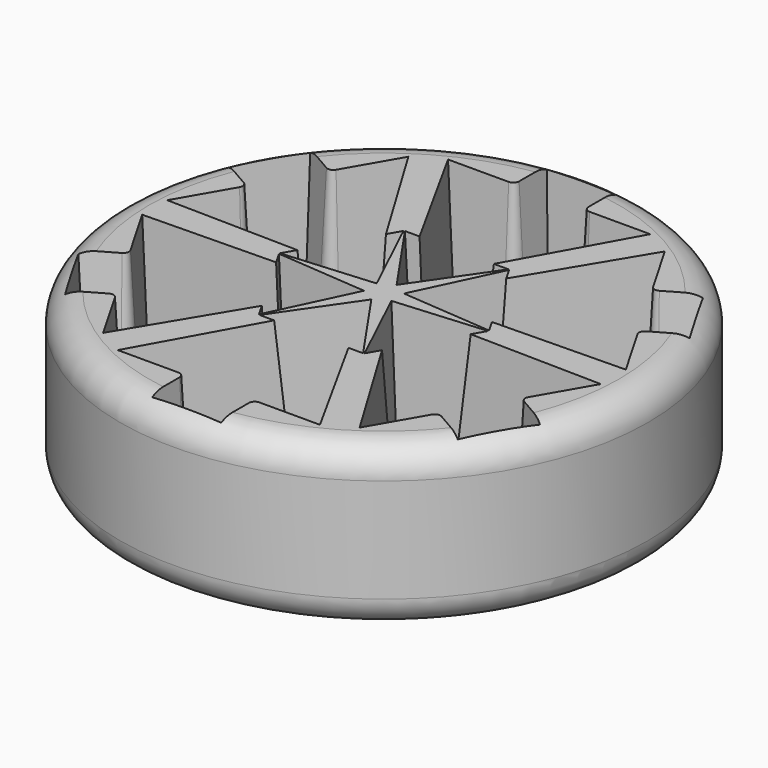
from build123d import *

# Parameters (mm, degrees)
F0_R            = 45.72
F1_DEPTH        = 28
F3_DEPTH        = 25.4
F3_TAPER        = 3
F3_COPIES_COUNT = 6
F5_R            = 1


# Not quite as in the source:
# - a fillet or chamfer that OpenCascade refuses, or shapes differently, is made with other operations: its cross-section is extruded or revolved along the edge and cut away or added
# - a pattern or mirror of a feature is missing from the dataset's text; its kind, count and spacing are read off the source's solid


with BuildPart() as f1:
    # F0 (on Top) → F1 (new body)
    with BuildSketch(Plane.XY):
        Circle(F0_R)
    extrude(amount=F1_DEPTH)

    # F2 (on face) → F3 (cut)
    with BuildSketch(Plane.XY.offset(28)):
        with BuildLine():
            Line((-6, -42.7338157296), (6, -42.7338157296))
            Line((6, -42.7338157296), (6, -36.7338157296))
            ThreePointArc((6, -36.7338157296), (6.2928932188, -36.0267089484), (7, -35.7338157296))
            Line((7, -35.7338157296), (17.5, -35.7338157296))
            Line((17.5, -35.7338157296), (6.4315567724, -15.7338157296))
            Line((6.4315567724, -15.7338157296), (8.9678969234, -15.7338157296))
            Line((8.9678969234, -15.7338157296), (0, -2.7338157296))
            Line((0, -2.7338157296), (-8.9678969234, -15.7338157296))
            Line((-8.9678969234, -15.7338157296), (-6.4315567724, -15.7338157296))
            Line((-6.4315567724, -15.7338157296), (-17.5, -35.7338157296))
            Line((-17.5, -35.7338157296), (-7, -35.7338157296))
            ThreePointArc((-7, -35.7338157296), (-6.2928932188, -36.0267089484), (-6, -36.7338157296))
            Line((-6, -36.7338157296), (-6, -42.7338157296))
        make_face()
    f3 = extrude(amount=-F3_DEPTH, taper=F3_TAPER, mode=Mode.SUBTRACT)

    # F3_copies: F3 ×6 about axis
    f3_copies_axis = Axis((0, 0, 0), (0, 0, 1))
    for i in range(1, F3_COPIES_COUNT):
        add(f3.rotate(f3_copies_axis, i * 360 / F3_COPIES_COUNT), mode=Mode.SUBTRACT)

    # F4: fillet of radius 5 on 2 edges, made by hand

    # F4_s1 → F4_t2 (revolve, cut)
    with BuildSketch(Plane.XZ):
        with BuildLine():
            ThreePointArc((45.72, 23), (44.2555339059, 26.5355339059), (40.72, 28))
            Line((40.72, 28), (45.72, 28))
            Line((45.72, 28), (45.72, 23))
        make_face()
    revolve(axis=Axis((0, 0, 28), (0, 0, 1)), mode=Mode.SUBTRACT)

    # F4_s3 → F4_t4 (revolve, cut)
    with BuildSketch(Plane.XZ):
        with BuildLine():
            ThreePointArc((45.72, 5), (44.2555339059, 1.4644660941), (40.72, 0))
            Line((40.72, 0), (45.72, 0))
            Line((45.72, 0), (45.72, 5))
        make_face()
    revolve(axis=Axis((0, 0, 0), (0, 0, 1)), mode=Mode.SUBTRACT)

    # F5
    f5_edges = [f1.edges().sort_by_distance(p)[0] for p in [
        (0, -41.402658, 2.6),
        (4.668842, -39.068237, 2.6),
        (5.351623, -35.085438, 2.6),
        (11.120948, -34.402658, 2.6),
        (9.707674, -24.402658, 2.6),
        (5.30295, -14.402658, 2.6),
        (3.216224, -9.740371, 2.6),
        (-3.216224, -9.740371, 2.6),
        (-5.30295, -14.402658, 2.6),
        (-9.707674, -24.402658, 2.6),
        (-11.120948, -34.402658, 2.6),
        (-5.351623, -35.085438, 2.6),
        (-4.668842, -39.068237, 2.6),
        (36.168507, 15.490782, 2.6),
        (35.855754, 20.701329, 2.6),
        (31.499664, 23.577455, 2.6),
        (4.668842, 39.068237, 2.6),
        (0, 41.402658, 2.6),
        (-4.668842, 39.068237, 2.6),
        (-31.499664, 23.577455, 2.6),
        (-35.855754, 20.701329, 2.6),
        (-36.168507, 15.490782, 2.6),
        (-36.168507, -15.490782, 2.6),
        (-35.855754, -20.701329, 2.6),
        (-31.499664, -23.577455, 2.6),
        (31.499664, -23.577455, 2.6),
        (35.855754, -20.701329, 2.6),
        (36.168507, -15.490782, 2.6),
        (-27.70907, -22.17736, 2.6),
        (-24.233102, -26.832352, 2.6),
        (-16.279485, -20.608421, 2.6),
        (-9.821593, -11.793819, 2.6),
        (-6.827297, -7.655517, 2.6),
        (-10.043521, -2.084854, 2.6),
        (-15.124543, -2.60884, 2.6),
        (-25.987159, -3.794237, 2.6),
        (-35.35405, -7.570306, 2.6),
        (-33.060692, -12.908078, 2.6),
        (-33.060692, 12.908078, 2.6),
        (-35.35405, 7.570306, 2.6),
        (-25.987159, 3.794237, 2.6),
        (-15.124543, 2.60884, 2.6),
        (-10.043521, 2.084854, 2.6),
        (-6.827297, 7.655517, 2.6),
        (-9.821593, 11.793819, 2.6),
        (-16.279485, 20.608421, 2.6),
        (-24.233102, 26.832352, 2.6),
        (-27.70907, 22.17736, 2.6),
        (-5.351623, 35.085438, 2.6),
        (-11.120948, 34.402658, 2.6),
        (-9.707674, 24.402658, 2.6),
        (-5.30295, 14.402658, 2.6),
        (-3.216224, 9.740371, 2.6),
        (3.216224, 9.740371, 2.6),
        (5.30295, 14.402658, 2.6),
        (9.707674, 24.402658, 2.6),
        (11.120948, 34.402658, 2.6),
        (5.351623, 35.085438, 2.6),
        (27.70907, 22.17736, 2.6),
        (24.233102, 26.832352, 2.6),
        (16.279485, 20.608421, 2.6),
        (9.821593, 11.793819, 2.6),
        (6.827297, 7.655517, 2.6),
        (10.043521, 2.084854, 2.6),
        (15.124543, 2.60884, 2.6),
        (25.987159, 3.794237, 2.6),
        (35.35405, 7.570306, 2.6),
        (33.060692, 12.908078, 2.6),
        (33.060692, -12.908078, 2.6),
        (35.35405, -7.570306, 2.6),
        (25.987159, -3.794237, 2.6),
        (15.124543, -2.60884, 2.6),
        (10.043521, -2.084854, 2.6),
        (6.827297, -7.655517, 2.6),
        (9.821593, -11.793819, 2.6),
        (16.279485, -20.608421, 2.6),
        (24.233102, -26.832352, 2.6),
        (27.70907, -22.17736, 2.6),
    ]]
    fillet(f5_edges, radius=F5_R)


solid = f1.part
